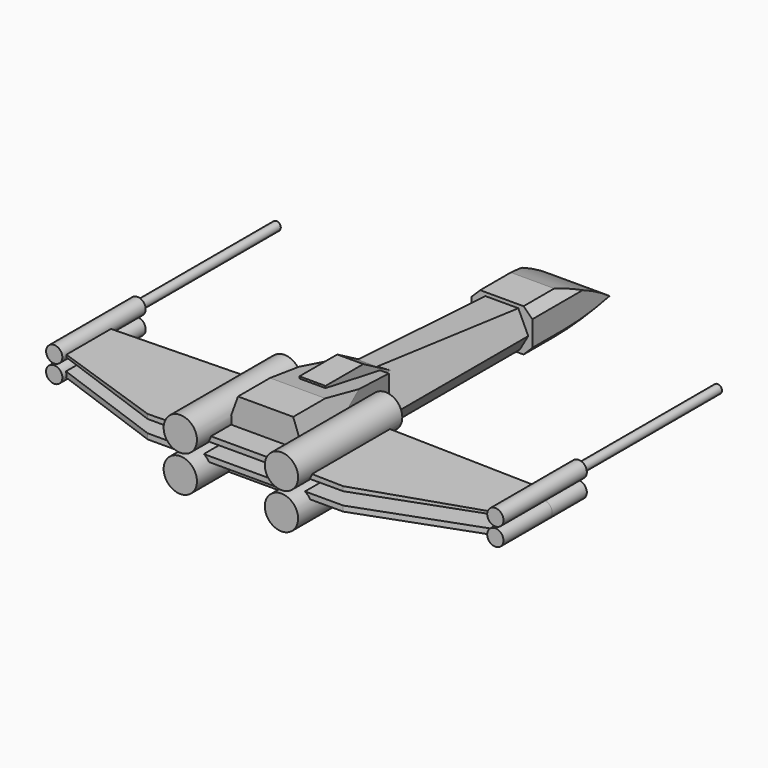
from build123d import *

# Parameters (mm, degrees)
F0_W           = 127.6564076543
F0_H           = 30.8224735782
F1_DEPTH       = 17.78
F2_SIZE2       = 7.3323484187
F2_SIZE        = 12.7
F3_T1_DEPTH    = 268.7880743195
F4_SIZE2       = 11.1110602678
F4_SIZE        = 127
F6_DEPTH       = 17.78
F7_SIZE        = 5.08
F8_SIZE        = 5.08
F9_W           = 74.2307901382
F9_H           = 40.582921356
F10_DEPTH      = 25.4
F11_SIZE2      = 8.95741062
F11_SIZE       = 50.8
F12_SIZE2      = 9.2448439504
F12_SIZE       = 25.4
F13_T4_DEPTH   = 389.5038855323
F13_T10_DEPTH  = 389.5038855323
F13_T16_DEPTH  = 389.5038855323
F14_SIZE2      = 58.064665698
F14_SIZE       = 5.08
F16_R          = 9.7471121544
F17_DEPTH      = 25.4
F17_DEPTH_BACK = 50.8
F18_W          = 57.0112913847
F18_H          = 3.1376983308
F19_DEPTH      = 127
F20_T4_DEPTH   = 585.328315574
F20_S5_R       = 9.7471121544
F20_T6_DEPTH   = 299
F21_SIZE2      = 69.7859264541
F21_SIZE       = 25.4
F21_2_SIZE2    = 69.7859264541
F21_2_SIZE     = 25.4
F23_R          = 4.7674452878
F24_DEPTH      = 25.4
F24_DEPTH_BACK = 35.56
F25_R          = 2.54
F27_DEPTH      = 101.6
F32_DEPTH      = 7.62
F32_DEPTH_BACK = 7.62


# Not quite as in the source:
# - a fillet or chamfer that OpenCascade refuses, or shapes differently, is made with other operations: its cross-section is extruded or revolved along the edge and cut away or added
# - a feature of the source that left no trace in its solid (it failed there, or was rolled back) is left out
# - a feature names something its author has since deleted; it is built from what else it names
# - the program builds the solid bodies; features that only make, move or delete a surface that nothing else refers to are left out


with BuildPart() as f1:
    # F0 (on Right) → F1 (new body)
    with BuildSketch(Plane.YZ):
        with Locations((-6.0360692441, 4.2380900122)):
            Rectangle(F0_W, F0_H)
    extrude(amount=F1_DEPTH)

    # F2
    f2_edges = [f1.edges().sort_by_distance(p)[0] for p in [
        (17.78, -6.036069, -11.173147),
    ]]
    f2_side = f1.faces().sort_by_distance((17.78, -6.036069, 4.23809))[0]
    chamfer(f2_edges, length=F2_SIZE, length2=F2_SIZE2, reference=f2_side)

    # F3: chamfer of 12.7 x 27.2352378905 on 1 edges, made by hand

    # F3_s2 → F3_t1 (cut)
    with BuildSketch(Plane.XZ.offset(-128.3579679156)):
        Polygon((17.78, -7.5859110892), (5.08, 19.6493268013), (17.78, 19.6493268013), align=None)
    extrude(amount=F3_T1_DEPTH, mode=Mode.SUBTRACT)

    # F4
    f4_edges = [f1.edges().sort_by_distance(p)[0] for p in [
        (2.54, 57.792135, 19.649327),
    ]]
    f4_side = f1.faces().sort_by_distance((2.54, -6.036069, 19.649327))[0]
    chamfer(f4_edges, length=F4_SIZE, length2=F4_SIZE2, reference=f4_side)

    # F5 (on Right) → F6 (join)
    with BuildSketch(Plane.YZ):
        with BuildLine():
            Line((64.5366609097, 11.9616184384), (42.1661399305, 11.9616184384))
            Line((42.1661399305, 11.9616184384), (42.1661399305, -12.9354065284))
            Line((42.1661399305, -12.9354065284), (64.5366609097, -12.9354065284))
            ThreePointArc((64.5366609097, -12.9354065284), (84.4675354935, -11.7221302623), (104.1040718555, -8.1002190709))
            ThreePointArc((104.1040718555, -8.1002190709), (85.3381650319, 3.9380759969), (64.5366609097, 11.9616184384))
        make_face()
    extrude(amount=F6_DEPTH)

    # F7
    f7_edges = [f1.edges().sort_by_distance(p)[0] for p in [
        (17.78, 53.3514, 11.961618),
    ]]
    chamfer(f7_edges, length=F7_SIZE)

    # F8
    f8_edges = [f1.edges().sort_by_distance(p)[0] for p in [
        (17.78, 53.3514, -12.935407),
    ]]
    chamfer(f8_edges, length=F8_SIZE)

    # F9 (on Right) → F10 (join)
    with BuildSketch(Plane.YZ):
        with Locations((-93.5413390398, 6.0360673815)):
            Rectangle(F9_W, F9_H)
    extrude(amount=F10_DEPTH)

    # F11
    f11_edges = [f1.edges().sort_by_distance(p)[0] for p in [
        (12.7, -56.425944, 26.327528),
    ]]
    f11_side = f1.faces().sort_by_distance((12.7, -93.541339, 26.327528))[0]
    chamfer(f11_edges, length=F11_SIZE, length2=F11_SIZE2, reference=f11_side)

    # F12
    f12_edges = [f1.edges().sort_by_distance(p)[0] for p in [
        (25.4, -118.941339, 26.327528),
    ]]
    f12_side = f1.faces().sort_by_distance((25.4, -95.190105, 4.622288))[0]
    chamfer(f12_edges, length=F12_SIZE, length2=F12_SIZE2, reference=f12_side)

    # F13: chamfer of 12.7 x 72.0252791091 on 1 edges, made by hand


with BuildPart() as f13_tool2:
    # F13_s3 → F13_t4 (new body)
    with BuildSketch(Plane.XY.offset(-201.4158753847)):
        Polygon((12.7, -56.4259439707), (25.4, -128.4512230798), (25.4, -56.4259439707), align=None)
    extrude(amount=F13_T4_DEPTH)

    split(bisect_by=Plane(origin=(11.6988093322, 0, 5.4552443829), x_dir=(0, 1, 0), z_dir=(-0.906307787, 0, -0.4226182617)), keep=Keep.TOP)

    split(bisect_by=Plane(origin=(12.6738531605, 0, -7.3172525339), x_dir=(0, 1, 0), z_dir=(0.8660254038, 0, -0.5)), keep=Keep.TOP)


with BuildPart() as f1_1:
    add(f1.part)

    # F13_t1: cut F13_tool2
    add(f13_tool2.part, mode=Mode.SUBTRACT)


with BuildPart() as f13_tool8:
    # F13_s9 → F13_t10 (new body)
    with BuildSketch(Plane.XY.offset(-201.4158753847)):
        Polygon((12.7, -56.4259439707), (25.4, -128.4512230798), (25.4, -56.4259439707), align=None)
    extrude(amount=F13_T10_DEPTH)

    split(bisect_by=Plane(origin=(11.6988093322, 0, 5.4552443829), x_dir=(0, 1, 0), z_dir=(0.906307787, 0, 0.4226182617)), keep=Keep.TOP)

    split(bisect_by=Plane(origin=(12.6738531605, 0, -7.3172525339), x_dir=(0, 1, 0), z_dir=(0.8660254038, 0, -0.5)), keep=Keep.TOP)


with BuildPart() as f1_2:
    add(f1_1.part)

    # F13_t7: cut F13_tool8
    add(f13_tool8.part, mode=Mode.SUBTRACT)


with BuildPart() as f13_tool14:
    # F13_s15 → F13_t16 (new body)
    with BuildSketch(Plane.XY.offset(-201.4158753847)):
        Polygon((12.7, -56.4259439707), (25.4, -128.4512230798), (25.4, -56.4259439707), align=None)
    extrude(amount=F13_T16_DEPTH)

    split(bisect_by=Plane(origin=(11.6988093322, 0, 5.4552443829), x_dir=(0, 1, 0), z_dir=(0.906307787, 0, 0.4226182617)), keep=Keep.TOP)

    split(bisect_by=Plane(origin=(12.6738531605, 0, -7.3172525339), x_dir=(0, 1, 0), z_dir=(-0.8660254038, 0, 0.5)), keep=Keep.TOP)


with BuildPart() as f1_3:
    add(f1_2.part)

    # F13_t13: cut F13_tool14
    add(f13_tool14.part, mode=Mode.SUBTRACT)

    # F14
    f14_edges = [f1_3.edges().sort_by_distance(p)[0] for p in [
        (6.35, -56.425944, -14.255393),
    ]]
    f14_side = f1_3.faces().sort_by_distance((6.915017, -56.425944, -12.427533))[0]
    chamfer(f14_edges, length=F14_SIZE, length2=F14_SIZE2, reference=f14_side)

    # F16 (on offset) → F17 (join, two sides)
    with BuildSketch(Plane.XZ.offset(130.6567341089)) as f17_sk:
        with Locations((29.5954812318, 13.0289848894)):
            Circle(F16_R)
        with Locations((29.5954812318, -8.2205578162)):
            Circle(F16_R)
    extrude(amount=F17_DEPTH)
    extrude(f17_sk.sketch, amount=-F17_DEPTH_BACK)

    # F18 (on Right) → F19 (join)
    with BuildSketch(Plane.YZ):
        with Locations((-116.8895885348, 8.9364784601)):
            Rectangle(F18_W, F18_H)
        with Locations((-116.8895885348, -1.5688491654)):
            Rectangle(F18_W, F18_H)
    extrude(amount=F19_DEPTH)

    # F20: chamfer of 101.6 x 1.7734345967 on 1 edges, made by hand


with BuildPart() as f20_tool2:
    # F20_s3 → F20_t4 (new body)
    with BuildSketch(Plane.XZ.offset(-175.7745692522)):
        Polygon((25.4, 10.5053276255), (127, 8.7318930288), (127, 10.5053276255), align=None)
    extrude(amount=F20_T4_DEPTH)

    # F20_s5 → F20_t6 (cut, symmetric)
    with BuildSketch(Plane.XZ.offset(116.9)):
        with Locations((29.5954812318, 13.0289848894)):
            Circle(F20_S5_R)
    extrude(amount=F20_T6_DEPTH, both=True, mode=Mode.SUBTRACT)


with BuildPart() as f1_4:
    add(f1_3.part)

    # F20_t1: cut F20_tool2
    add(f20_tool2.part, mode=Mode.SUBTRACT)

    # F21
    f21_edges = [f1_4.edges().sort_by_distance(p)[0] for p in [
        (127, -145.395234, 8.049761),
    ]]
    f21_side = f1_4.faces().sort_by_distance((127, -116.889589, 8.049761))[0]
    chamfer(f21_edges, length=F21_SIZE, length2=F21_SIZE2, reference=f21_side)

    # F21#2
    f21_2_edges = [f1_4.edges().sort_by_distance(p)[0] for p in [
        (127, -145.395234, -1.568849),
    ]]
    f21_2_side = f1_4.faces().sort_by_distance((127, -116.889589, -1.568849))[0]
    chamfer(f21_2_edges, length=F21_2_SIZE, length2=F21_2_SIZE2, reference=f21_2_side)

    # F23 (on offset) → F24 (join, two sides)
    with BuildSketch(Plane(origin=(0, -88.3839428425, 0), x_dir=(-1, 0, 0), z_dir=(0, 1, 0))) as f24_sk:
        with Locations((-129.0663182735, 8.6347437004)):
            Circle(F23_R)
        with Locations((-129.0663182735, -1.823012135)):
            Circle(F23_R)
    extrude(amount=F24_DEPTH)
    extrude(f24_sk.sketch, amount=-F24_DEPTH_BACK)

    # F29: F1, F27 across plane


with BuildPart() as f27:
    # F25 (on face) → F27 (new body)
    with BuildSketch(Plane(origin=(0, -62.9839428425, 0), x_dir=(-1, 0, 0), z_dir=(0, 1, 0))):
        with Locations((-129.0663182735, 8.6347437004)):
            Circle(F25_R)
    extrude(amount=F27_DEPTH)


with BuildPart() as f1_5:
    add(f1_4.part)
    add(f1_4.part.mirror(Plane.YZ))
    add(f27.part.mirror(Plane.YZ))

    # F31 (on Right) → F32 (join, two sides)
    with BuildSketch(Plane.YZ) as f32_sk:
        Polygon((-68.7129795551, 25.559393689), (-96.3866710663, 25.559393689), (-96.3866710663, 4.902585643), (-68.7129795551, 4.902585643), (-34.1929905117, 6.0028838925), align=None)
    extrude(amount=F32_DEPTH)
    extrude(f32_sk.sketch, amount=-F32_DEPTH_BACK)


solid = Compound([f27.part, f1_5.part])
